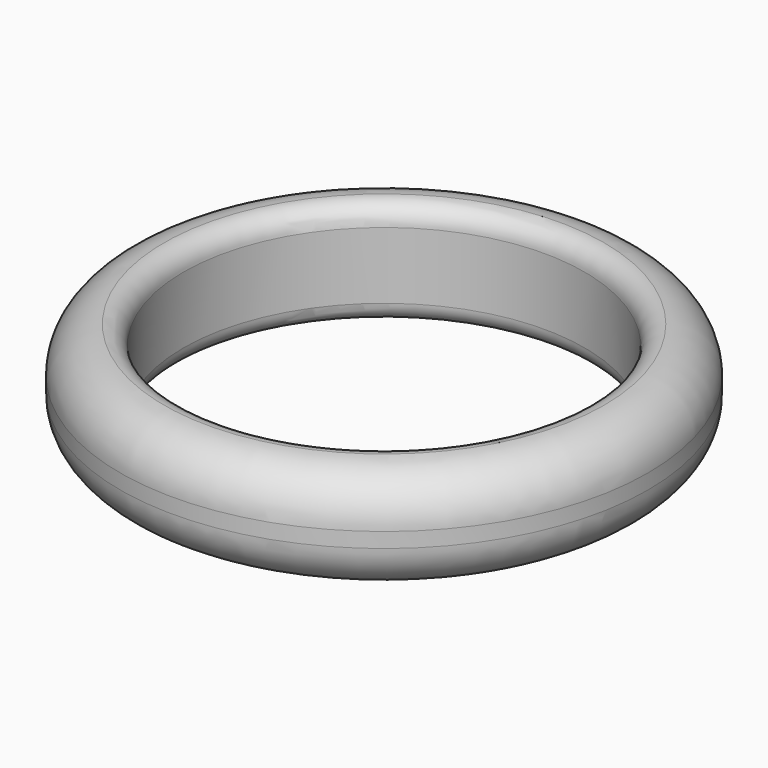
from build123d import *

# Parameters (mm, degrees)
F0_R     = 12.5
F0_R_2   = 9.5
F1_DEPTH = 5
F2_R     = 0.9198153673


# Not quite as in the source:
# - a fillet or chamfer that OpenCascade refuses, or shapes differently, is made with other operations: its cross-section is extruded or revolved along the edge and cut away or added


with BuildPart() as f1:
    # F0 (on Top) → F1 (new body)
    with BuildSketch(Plane.XY):
        Circle(F0_R)
        Circle(F0_R_2, mode=Mode.SUBTRACT)
    extrude(amount=F1_DEPTH)

    # F2
    f2_edges = [f1.edges().sort_by_distance(p)[0] for p in [
        (-9.5, 0, 5),
        (-9.5, 0, 0),
    ]]
    fillet(f2_edges, radius=F2_R)

    # F3: fillet of radius 2.1462358569 on 2 edges, made by hand

    # F3_s1 → F3_t2 (revolve, cut)
    with BuildSketch(Plane.XZ):
        with BuildLine():
            ThreePointArc((10.4198153673, 0), (11.8945577469, 0.6511364368), (12.5, 2.1452192404))
            Line((12.5, 2.1452192404), (12.5429247171, 2.1452192404))
            Line((12.5429247171, 2.1452192404), (12.5429247171, 0))
            Line((12.5429247171, 0), (12.5, -0.0429247171))
            ThreePointArc((12.5, -0.0429247171), (11.4599076836, -0.0429247171), (10.4211363917, -0.0429043848))
            Line((10.4211363917, -0.0429043848), (10.4198153673, 0))
        make_face()
    revolve(axis=Axis((0, 0, 0), (0, 0, 1)), mode=Mode.SUBTRACT)

    # F3_s3 → F3_t4 (revolve, cut)
    with BuildSketch(Plane.XZ):
        with BuildLine():
            ThreePointArc((10.4198153673, 5), (11.8945577469, 4.3488635632), (12.5, 2.8547807596))
            Line((12.5, 2.8547807596), (12.5429247171, 2.8547807596))
            Line((12.5429247171, 2.8547807596), (12.5429247171, 5))
            Line((12.5429247171, 5), (12.5, 5.0429247171))
            ThreePointArc((12.5, 5.0429247171), (11.4599076836, 5.0429247171), (10.4211363917, 5.0429043848))
            Line((10.4211363917, 5.0429043848), (10.4198153673, 5))
        make_face()
    revolve(axis=Axis((0, 0, 5), (0, 0, 1)), mode=Mode.SUBTRACT)


solid = f1.part
